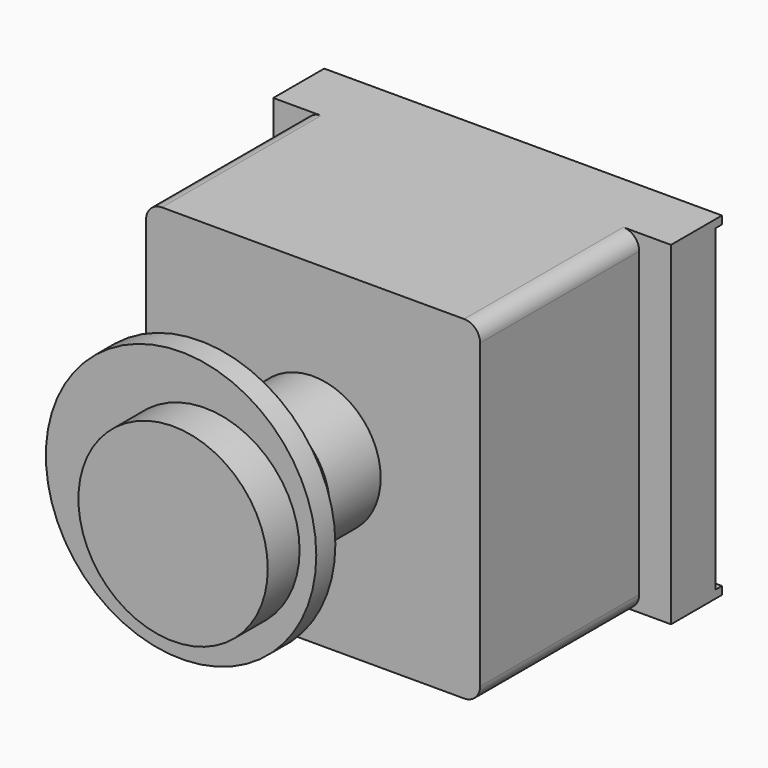
from build123d import *

# Parameters (mm, degrees)
F0_R      = 26.9875
F0_R_2    = 19.3675
F1_DEPTH  = 25.4
F2_DEPTH  = 79.375
F3_DEPTH  = 44.45
F4_R      = 37.792391803
F4_R_2    = 28.575
F4_R_3    = 19.3675
F5_DEPTH  = 25.4
F4_R_4    = 53.975
F6_DEPTH  = 9.525
F7_DEPTH  = 19.05
F8_DEPTH  = 19.05
F9_R      = 19.3675
F10_DEPTH = 22.225
F11_W     = 3.175
F11_H     = 3.175
F12_DEPTH = 158.75


with BuildPart() as f1:
    # F0 (on Front) → F1 (new body)
    with BuildSketch(Plane.XZ):
        with Locations((-66.675, 66.675)):
            Circle(F0_R)
        with Locations((-66.675, 66.675)):
            Circle(F0_R_2, mode=Mode.SUBTRACT)
    extrude(amount=F1_DEPTH)

    # F0 (on Front) → F2 (join)
    with BuildSketch(Plane.XZ):
        with BuildLine():
            Line((-127, 0), (-6.35, 0))
            ThreePointArc((-6.35, 0), (-1.8598719395, 1.8598719395), (0, 6.35))
            Line((0, 6.35), (0, 127))
            ThreePointArc((0, 127), (-1.8598719395, 131.4901280605), (-6.35, 133.35))
            Line((-6.35, 133.35), (-127, 133.35))
            ThreePointArc((-127, 133.35), (-131.4901280605, 131.4901280605), (-133.35, 127))
            Line((-133.35, 127), (-133.35, 6.35))
            ThreePointArc((-133.35, 6.35), (-131.4901280605, 1.8598719395), (-127, 0))
        make_face()
        with Locations((-66.675, 66.675)):
            Circle(F0_R, mode=Mode.SUBTRACT)
        with Locations((-66.675, 66.675)):
            Circle(F0_R)
        with Locations((-66.675, 66.675)):
            Circle(F0_R_2, mode=Mode.SUBTRACT)
    extrude(amount=-F2_DEPTH)

    # F9 (on face) → F10 (join)
    with BuildSketch(Plane(origin=(0, 79.375, 0), x_dir=(-1, 0, 0), z_dir=(0, 1, 0))):
        with BuildLine():
            Line((6.35, 133.35), (-12.7, 133.35))
            Line((-12.7, 133.35), (-12.7, 0))
            Line((-12.7, 0), (6.35, 0))
            ThreePointArc((6.35, 0), (1.8598719395, 1.8598719395), (0, 6.35))
            Line((0, 6.35), (0, 127))
            ThreePointArc((0, 127), (1.8598719395, 131.4901280605), (6.35, 133.35))
        make_face()
        with BuildLine():
            Line((127, 133.35), (6.35, 133.35))
            ThreePointArc((6.35, 133.35), (1.8598719395, 131.4901280605), (0, 127))
            Line((0, 127), (0, 6.35))
            ThreePointArc((0, 6.35), (1.8598719395, 1.8598719395), (6.35, 0))
            Line((6.35, 0), (127, 0))
            ThreePointArc((127, 0), (131.4901280605, 1.8598719395), (133.35, 6.35))
            Line((133.35, 6.35), (133.35, 127))
            ThreePointArc((133.35, 127), (131.4901280605, 131.4901280605), (127, 133.35))
        make_face()
        with Locations((66.675, 66.675)):
            Circle(F9_R, mode=Mode.SUBTRACT)
        with BuildLine():
            Line((146.05, 133.35), (127, 133.35))
            ThreePointArc((127, 133.35), (131.4901280605, 131.4901280605), (133.35, 127))
            Line((133.35, 127), (133.35, 6.35))
            ThreePointArc((133.35, 6.35), (131.4901280605, 1.8598719395), (127, 0))
            Line((127, 0), (146.05, 0))
            Line((146.05, 0), (146.05, 133.35))
        make_face()
        with Locations((66.675, 66.675)):
            Circle(F9_R)
    extrude(amount=F10_DEPTH)

    # F11 (on face) → F12 (join)
    with BuildSketch(Plane(origin=(-146.05, 0, 0), x_dir=(0, -1, 0), z_dir=(-1, 0, 0))):
        with Locations((-103.1875, 131.7625)):
            Rectangle(F11_W, F11_H)
        with Locations((-103.1875, 1.5875)):
            Rectangle(F11_W, F11_H)
    extrude(amount=-F12_DEPTH)


with BuildPart() as f3:
    # F0 (on Front) → F3 (new body, symmetric)
    with BuildSketch(Plane.XZ):
        with Locations((-66.675, 66.675)):
            Circle(F0_R_2)
    extrude(amount=F3_DEPTH, both=True)

    # F4 (on face) → F8 (join)
    with BuildSketch(Plane.XZ.offset(44.45)):
        with Locations((-66.675, 66.675)):
            Circle(F4_R_3)
    extrude(amount=F8_DEPTH)


with BuildPart() as f5:
    # F4 (on face) → F5 (new body)
    with BuildSketch(Plane.XZ.offset(44.45)):
        with Locations((-66.675, 66.675)):
            Circle(F4_R)
        with Locations((-66.675, 66.675)):
            Circle(F4_R_2, mode=Mode.SUBTRACT)
        with Locations((-66.675, 66.675)):
            Circle(F4_R_2)
        with Locations((-66.675, 66.675)):
            Circle(F4_R_3, mode=Mode.SUBTRACT)
        with Locations((-66.675, 66.675)):
            Circle(F4_R_3)
    extrude(amount=F5_DEPTH)

    # F4 (on face) → F6 (join)
    with BuildSketch(Plane.XZ.offset(44.45)):
        with Locations((-76.1897387261, 67.1170090193)):
            Circle(F4_R_4)
        with Locations((-66.675, 66.675)):
            Circle(F4_R, mode=Mode.SUBTRACT)
    extrude(amount=F6_DEPTH)

    # F4 (on face) → F7 (cut)
    with BuildSketch(Plane.XZ.offset(44.45)):
        with Locations((-66.675, 66.675)):
            Circle(F4_R_2)
        with Locations((-66.675, 66.675)):
            Circle(F4_R_3, mode=Mode.SUBTRACT)
        with Locations((-66.675, 66.675)):
            Circle(F4_R_3)
    extrude(amount=F7_DEPTH, mode=Mode.SUBTRACT)


solid = Compound([f1.part, f3.part, f5.part])
